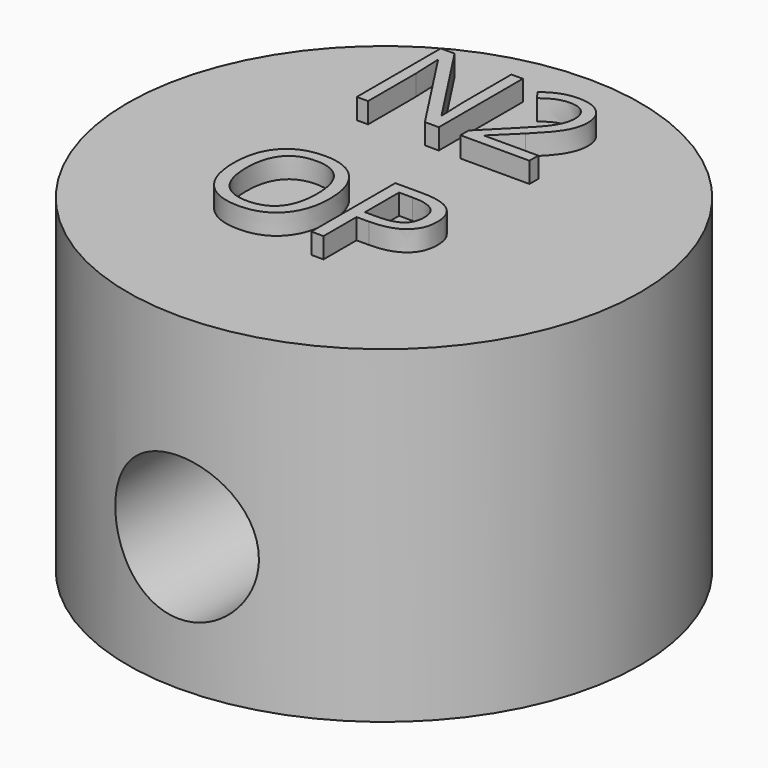
from build123d import *

# Parameters (mm, degrees)
F0_R         = 12.5
F1_DEPTH     = 16
F3_R         = 3.5
F4_DEPTH     = 25.001
F5_TEXT_SIZE = 7.171671896
F6_DEPTH     = 1


# Not quite as in the source:
# - Text() gives the source's letters only with a copy of the font that has no kerning and outlines rounded to 1/6400 em; it was checked with that copy


with BuildPart() as f1:
    # F0 (on Top) → F1 (new body)
    with BuildSketch(Plane.XY):
        Circle(F0_R)
    extrude(amount=F1_DEPTH)

    # F3 (on offset) → F4 (cut, through all)
    with BuildSketch(Plane.XZ.offset(-12.5)):
        with Locations((0, 6.5)):
            Circle(F3_R)
    extrude(amount=F4_DEPTH, mode=Mode.SUBTRACT)

    # F5 (on face) → F6 (join)
    with BuildSketch(Plane.XY.offset(16)):
        with Locations((-5.5, 4.3363962349)):
            Text('N2', F5_TEXT_SIZE, font='Open Sans', text_align=(TextAlign.LEFT, TextAlign.BOTTOM))
        with Locations((-5.5, -5.4170775437)):
            Text('OP', F5_TEXT_SIZE, font='Open Sans', text_align=(TextAlign.LEFT, TextAlign.BOTTOM))
    extrude(amount=F6_DEPTH)


solid = f1.part
